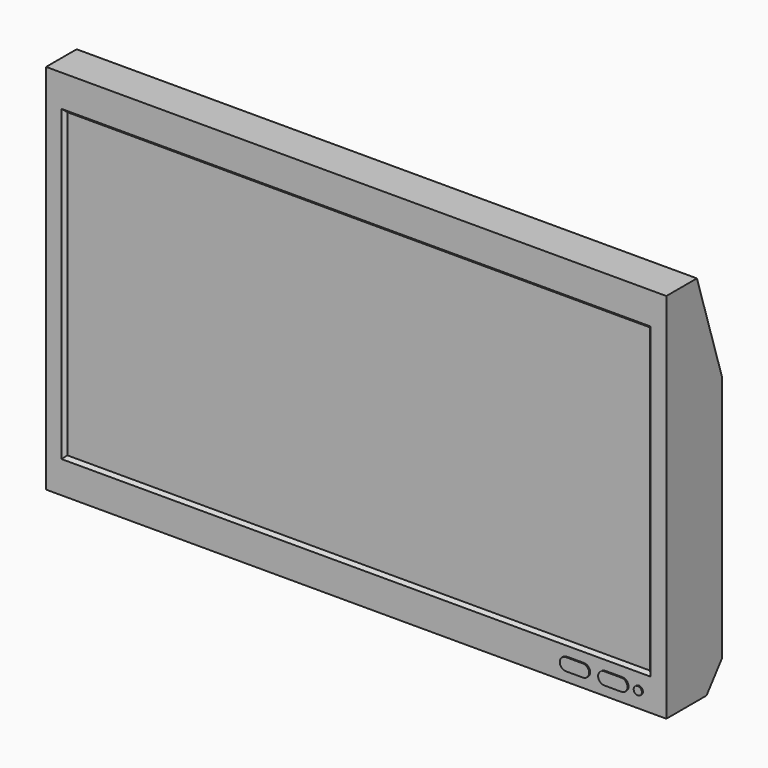
from build123d import *

# Parameters (mm, degrees)
F1_DEPTH     = 317.5
F2_W         = 606.8687809474
F2_H         = 319.4243614871
F3_DEPTH     = 3.175
F4_T4_DEPTH  = 345.5526606448
F4_T9_DEPTH  = 632.9970801051
F4_T14_DEPTH = 345.5526606448
F4_T19_DEPTH = 632.9970801051
F5_R         = 4.2314330569
F6_DEPTH     = 1.27


# Not quite as in the source:
# - a fillet or chamfer that OpenCascade refuses, or shapes differently, is made with other operations: its cross-section is extruded or revolved along the edge and cut away or added


with BuildPart() as f1:
    # F0 (on Right) → F1 (new body, symmetric)
    with BuildSketch(Plane.YZ):
        Polygon((0, 381), (0, 0), (51.4319166541, 0), (71.12, 25.4), (71.12, 279.4), (39.1150377691, 381), align=None)
    extrude(amount=F1_DEPTH, both=True)

    # F2 (on face) → F3 (cut)
    with BuildSketch(Plane.XZ):
        with Locations((0, 190.5)):
            Rectangle(F2_W, F2_H)
    extrude(amount=-F3_DEPTH, mode=Mode.SUBTRACT)

    # F4: chamfer of 5.08 on 4 edges, made by hand


with BuildPart() as f4_tool2:
    # F4_s3 → F4_t4 (new body)
    with BuildSketch(Plane.XY.offset(363.2763303224)):
        Polygon((-303.4343904737, -1.905), (-298.3543904737, 3.175), (-303.4343904737, 3.175), align=None)
    extrude(amount=-F4_T4_DEPTH)

    split(bisect_by=Plane.XZ, keep=Keep.BOTTOM)


with BuildPart() as f1_1:
    add(f1.part)

    # F4_t1: union F4_tool2
    add(f4_tool2.part)


with BuildPart() as f4_tool7:
    # F4_s8 → F4_t9 (new body)
    with BuildSketch(Plane.YZ.offset(316.4985400526)):
        Polygon((-1.905, 350.2121807435), (3.175, 345.1321807435), (3.175, 350.2121807435), align=None)
    extrude(amount=-F4_T9_DEPTH)

    split(bisect_by=Plane.XZ, keep=Keep.BOTTOM)


with BuildPart() as f1_2:
    add(f1_1.part)

    # F4_t6: union F4_tool7
    add(f4_tool7.part)


with BuildPart() as f4_tool12:
    # F4_s13 → F4_t14 (new body)
    with BuildSketch(Plane.XY.offset(17.7236696776)):
        Polygon((303.4343904737, -1.905), (298.3543904737, 3.175), (303.4343904737, 3.175), align=None)
    extrude(amount=F4_T14_DEPTH)

    split(bisect_by=Plane.XZ, keep=Keep.BOTTOM)


with BuildPart() as f1_3:
    add(f1_2.part)

    # F4_t11: union F4_tool12
    add(f4_tool12.part)


with BuildPart() as f4_tool17:
    # F4_s18 → F4_t19 (new body)
    with BuildSketch(Plane.YZ.offset(-316.4985400526)):
        Polygon((-1.905, 30.7878192565), (3.175, 35.8678192565), (3.175, 30.7878192565), align=None)
    extrude(amount=F4_T19_DEPTH)

    split(bisect_by=Plane.XZ, keep=Keep.BOTTOM)


with BuildPart() as f1_4:
    add(f1_3.part)

    # F4_t16: union F4_tool17
    add(f4_tool17.part)

    # F5 (on face) → F6 (join)
    with BuildSketch(Plane.XZ):
        with BuildLine():
            ThreePointArc((233.1511284661, 10.1901956652), (239.5011284661, 16.5401956652), (233.1511284661, 22.8901956652))
            Line((233.1511284661, 22.8901956652), (215.7576586556, 22.8901956652))
            ThreePointArc((215.7576586556, 22.8901956652), (209.4076586556, 16.5401956652), (215.7576586556, 10.1901956652))
            Line((215.7576586556, 10.1901956652), (233.1511284661, 10.1901956652))
        make_face()
        with BuildLine():
            ThreePointArc((272.4028527737, 10.1901956652), (278.7528527737, 16.5401956652), (272.4028527737, 22.8901956652))
            Line((272.4028527737, 22.8901956652), (255.0093829632, 22.8901956652))
            ThreePointArc((255.0093829632, 22.8901956652), (248.6593829632, 16.5401956652), (255.0093829632, 10.1901956652))
            Line((255.0093829632, 10.1901956652), (272.4028527737, 10.1901956652))
        make_face()
        with Locations((289.2993986607, 16.5401956652)):
            Circle(F5_R)
    extrude(amount=F6_DEPTH)


solid = f1_4.part
